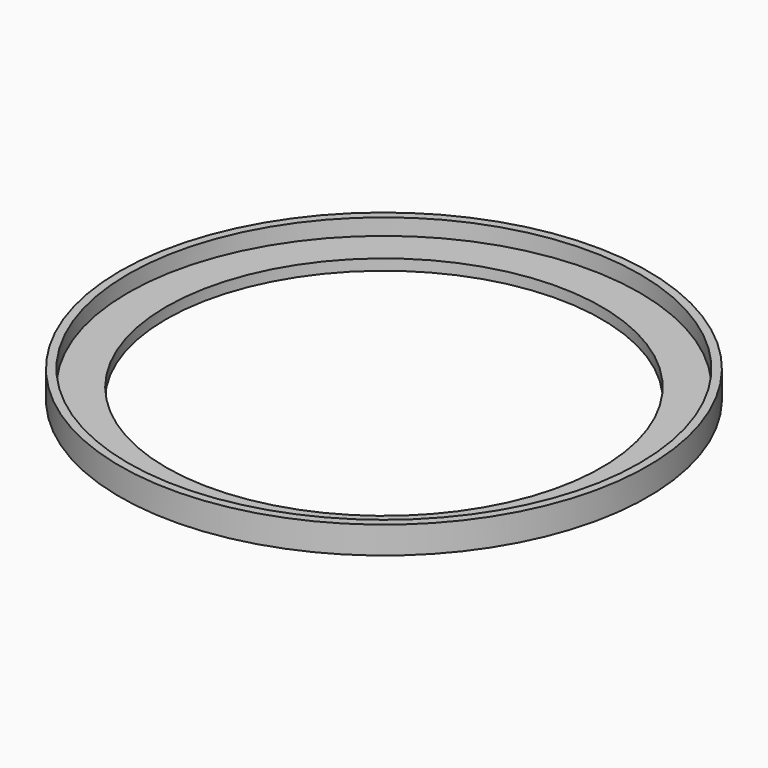
from build123d import *


# Not quite as in the source:
# - ends of sketch curves that miss each other by under 0.0002 mm in the source are joined


with BuildPart() as f1:
    # F0 (on Front) → F1 (revolve)
    with BuildSketch(Plane.XZ):
        Polygon((-80, 3), (-94, 3), (-93.9999967813, 9), (-97.000002861, 9), (-97.000002861, 3), (-97, -1), (-80, -1), align=None)
    revolve(axis=Axis((0, 0, 1.5), (0, 0, -1)))


solid = f1.part
